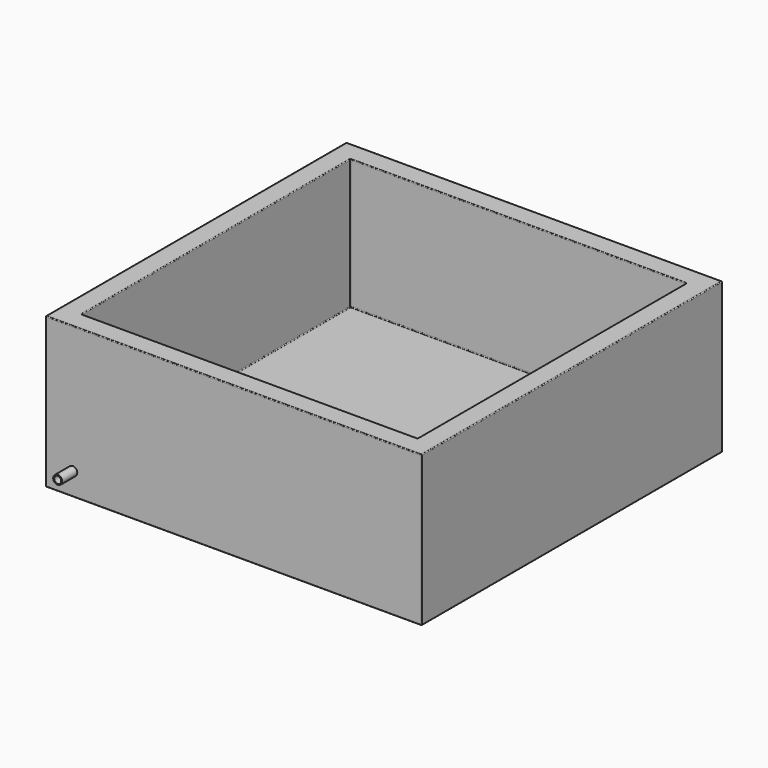
from build123d import *

# Parameters (mm, degrees)
F0_W           = 500
F0_H           = 500
F1_DEPTH       = 200
F2_R           = 1
F3_T           = -1.6
F4_W           = 496.8
F4_H           = 496.8
F4_W_2         = 450
F4_H_2         = 450
F5_DEPTH       = 1.6
F6_W           = 450
F6_H           = 450
F7_DEPTH       = 175
F8_T           = 1.6
F8_T3_DEPTH    = 453.2
F8_T5_DEPTH    = 453.2
F9_R           = 1
F9_2_R         = 1
F10_R          = 6
F11_DEPTH      = 25
F12_R          = 6
F13_DEPTH      = 25
F14_R          = 4.6271608876
F15_DEPTH      = 30
F16_R          = 4.4168784141
F17_DEPTH      = 30
F18_R          = 6
F19_DEPTH      = 26.6
F19_DEPTH_BACK = 25
F20_R          = 4.5305063865
F21_DEPTH      = 70


# Not quite as in the source:
# - a shell that OpenCascade refuses in one call is made with other operations: the cavity is built on its own and cut out


with BuildPart() as f1:
    # F0 (on Top) → F1 (new body)
    with BuildSketch(Plane.XY):
        Rectangle(F0_W, F0_H)
    extrude(amount=F1_DEPTH)

    # F2
    f2_edges = [f1.edges().sort_by_distance(p)[0] for p in [
        (250, 0, 0),
        (0, 250, 0),
        (-250, 0, 0),
        (0, -250, 0),
        (250, -250, 100),
        (-250, -250, 100),
        (-250, 250, 100),
        (250, 250, 100),
    ]]
    fillet(f2_edges, radius=F2_R)

    # F3
    f3_openings = [f1.faces().sort_by_distance(p)[0] for p in [
        (0, 0, 200),
    ]]
    offset(amount=F3_T, openings=f3_openings)

    # F9#2
    f9_2_edges = [f1.edges().sort_by_distance(p)[0] for p in [
        (-250, 0, 200),
        (0, -250, 200),
        (250, 0, 200),
        (0, 250, 200),
    ]]
    fillet(f9_2_edges, radius=F9_2_R)


with BuildPart() as f5:
    # F4 (on face) → F5 (new body)
    with BuildSketch(Plane.XY.offset(200)):
        Rectangle(F4_W, F4_H)
        Rectangle(F4_W_2, F4_H_2, mode=Mode.SUBTRACT)
    extrude(amount=-F5_DEPTH)

    # F6 (on face) → F7 (join)
    with BuildSketch(Plane.XY.offset(200)):
        Rectangle(F6_W, F6_H)
    extrude(amount=-F7_DEPTH)

    # F8: shell of thickness 1.6, made by hand


with BuildPart() as f8_core1:
    # F8_t2: copy of F5
    add(f5.part)

    # the walls: a layer under each face that stays
    f8_faces = [f8_core1.faces().sort_by_distance(p)[0] for p in [
        (248.4, 0, 199.2),
        (0, -248.4, 199.2),
        (0, 248.4, 199.2),
        (-231.84, -231.84, 198.4),
        (-248.4, 0, 199.2),
        (-225, 0, 111.7),
        (0, 225, 111.7),
        (225, 0, 111.7),
        (0, -225, 111.7),
        (0, 0, 25),
    ]]
    thicken(f8_faces, amount=-F8_T, mode=Mode.SUBTRACT)

    # F8_s4 → F8_t3 (cut)
    with BuildSketch(Plane.XZ.offset(-226.6)):
        Polygon((-225.016, 198.384), (-225, 200), (-223.4, 200), (-223.4, 198.4), align=None)
        Polygon((225.016, 198.384), (225, 200), (223.4, 200), (223.4, 198.4), align=None)
    extrude(amount=F8_T3_DEPTH, mode=Mode.SUBTRACT)

    # F8_s6 → F8_t5 (cut)
    with BuildSketch(Plane.YZ.offset(-226.6)):
        Polygon((225.016, 198.384), (225, 200), (223.4, 200), (223.4, 198.4), align=None)
        Polygon((-225.016, 198.384), (-225, 200), (-223.4, 200), (-223.4, 198.4), align=None)
    extrude(amount=F8_T5_DEPTH, mode=Mode.SUBTRACT)


with BuildPart() as f5_1:
    add(f5.part)

    # what is left inside the walls is the cavity
    f8_cavity = [f8_core1.part.solids().sort_by_distance(p)[0] for p in [
        (0, -74.466667, 199.984),
    ]]
    add(f8_cavity, mode=Mode.SUBTRACT)

    # F9
    f9_edges = [f5_1.edges().sort_by_distance(p)[0] for p in [
        (-223.4, 0, 200),
        (0, -223.4, 200),
        (0, 223.4, 200),
        (223.4, 0, 200),
        (-223.4, 223.4, 113.3),
        (0, 223.4, 26.6),
        (223.4, 0, 26.6),
        (0, -223.4, 26.6),
        (-223.4, 0, 26.6),
        (223.4, -223.4, 113.3),
        (-223.4, -223.4, 113.3),
        (223.4, 223.4, 113.3),
    ]]
    fillet(f9_edges, radius=F9_R)


with BuildPart() as f11:
    # F10 (on face) → F11 (new body)
    with BuildSketch(Plane(origin=(0, 250, 0), x_dir=(-1, 0, 0), z_dir=(0, 1, 0))):
        with Locations((-220, 170)):
            Circle(F10_R)
    extrude(amount=F11_DEPTH)


with BuildPart() as f13:
    # F12 (on face) → F13 (new body)
    with BuildSketch(Plane.XZ.offset(250)):
        with Locations((-214, 30)):
            Circle(F12_R)
    extrude(amount=F13_DEPTH)


with BuildPart() as f15_tool:
    # F14 (on face) → F15 (new body)
    with BuildSketch(Plane.XZ.offset(275)):
        with Locations((-214, 30)):
            Circle(F14_R)
    extrude(amount=-F15_DEPTH)


with BuildPart() as f1_1:
    add(f1.part)

    # F15: cut by f15_tool
    add(f15_tool.part, mode=Mode.SUBTRACT)


with BuildPart() as f13_1:
    add(f13.part)

    # F15: cut by f15_tool
    add(f15_tool.part, mode=Mode.SUBTRACT)


with BuildPart() as f17_tool:
    # F16 (on face) → F17 (new body)
    with BuildSketch(Plane(origin=(0, 275, 0), x_dir=(-1, 0, 0), z_dir=(0, 1, 0))):
        with Locations((-220, 170)):
            Circle(F16_R)
    extrude(amount=-F17_DEPTH)


with BuildPart() as f1_2:
    add(f1_1.part)

    # F17: cut by f17_tool
    add(f17_tool.part, mode=Mode.SUBTRACT)


with BuildPart() as f11_1:
    add(f11.part)

    # F17: cut by f17_tool
    add(f17_tool.part, mode=Mode.SUBTRACT)


with BuildPart() as f19:
    # F18 (on face) → F19 (new body, two sides)
    with BuildSketch(Plane(origin=(0, 250, 0), x_dir=(-1, 0, 0), z_dir=(0, 1, 0))) as f19_sk:
        with Locations((-135.3337168694, 31.1506576836)):
            Circle(F18_R)
    extrude(amount=-F19_DEPTH)
    extrude(f19_sk.sketch, amount=F19_DEPTH_BACK)


with BuildPart() as f21_tool:
    # F20 (on face) → F21 (new body)
    with BuildSketch(Plane(origin=(0, 275, 0), x_dir=(-1, 0, 0), z_dir=(0, 1, 0))):
        with Locations((-135.3337168694, 31.1506576836)):
            Circle(F20_R)
    extrude(amount=-F21_DEPTH)


with BuildPart() as f1_3:
    add(f1_2.part)

    # F21: cut by f21_tool
    add(f21_tool.part, mode=Mode.SUBTRACT)


with BuildPart() as f5_2:
    add(f5_1.part)

    # F21: cut by f21_tool
    add(f21_tool.part, mode=Mode.SUBTRACT)


with BuildPart() as f19_1:
    add(f19.part)

    # F21: cut by f21_tool
    add(f21_tool.part, mode=Mode.SUBTRACT)


solid = Compound([f13_1.part, f11_1.part, f1_3.part, f5_2.part, f19_1.part])
